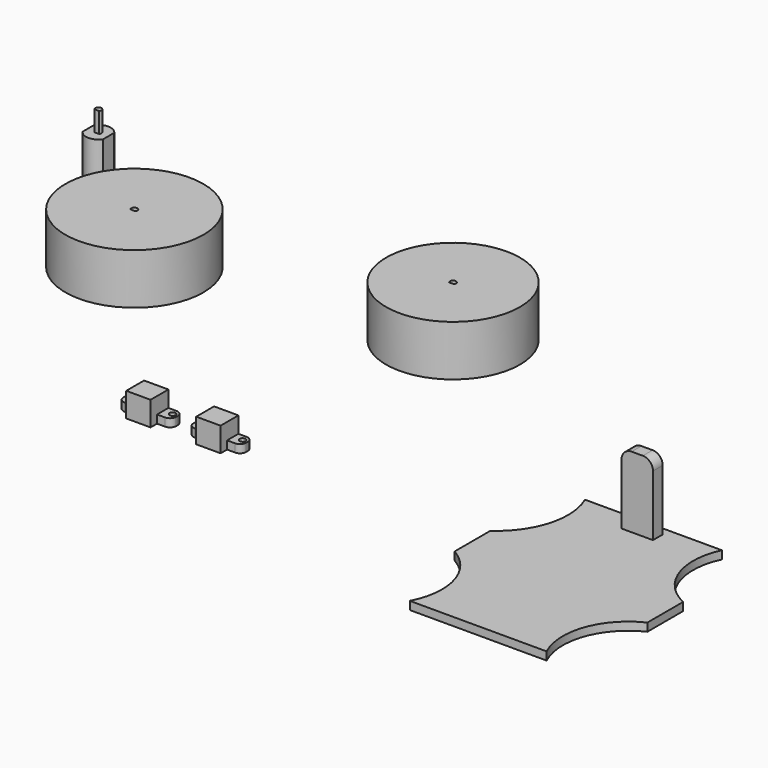
from build123d import *

# Parameters (mm, degrees)
F0_R      = 34
F1_DEPTH  = 25
F4_DEPTH  = 44
F5_DEPTH  = 25
F7_DEPTH  = 10
F8_R      = 33
F9_DEPTH  = 25
F11_DEPTH = 28.1
F13_W     = 95
F13_H     = 108
F14_DEPTH = 4
F16_DEPTH = 25
F17_W     = 15.5
F17_H     = 6
F18_DEPTH = 35
F19_R     = 5
F21_DEPTH = 12
F22_W     = 7
F22_H     = 7
F23_DEPTH = 8
F24_R     = 3
F26_R     = 1.5
F25_R     = 1.5
F27_DEPTH = 25
F29_DEPTH = 12
F30_W     = 7
F30_H     = 7
F31_DEPTH = 8
F32_R     = 3
F33_R     = 3
F34_R     = 1.5
F35_R     = 1.5
F36_DEPTH = 25


with BuildPart() as f1:
    # F0 (on Top) → F1 (new body)
    with BuildSketch(Plane.XY):
        Circle(F0_R)
    extrude(amount=F1_DEPTH)

    # F3 (on face) → F4 (cut)
    with BuildSketch(Plane.XY.offset(25)):
        with BuildLine():
            Line((0, -1), (1.1180339887, -1))
            ThreePointArc((1.1180339887, -1), (0, 1.5), (-1.1180339887, -1))
            Line((-1.1180339887, -1), (0, -1))
        make_face()
    extrude(amount=-F4_DEPTH, mode=Mode.SUBTRACT)


with BuildPart() as f5:
    # F2 (on Top) → F5 (new body)
    with BuildSketch(Plane.XY):
        with BuildLine():
            Line((-56.0500432012, 44.9939276846), (-56.0500432012, 38.1657885869))
            ThreePointArc((-56.0500432012, 38.1657885869), (-50.9907110945, 35.4763581357), (-45.9313789879, 38.1657885869))
            Line((-45.9313789879, 38.1657885869), (-45.9313789879, 44.9939276846))
            ThreePointArc((-45.9313789879, 44.9939276846), (-50.9907110945, 47.6833581357), (-56.0500432012, 44.9939276846))
        make_face()
    extrude(amount=F5_DEPTH)

    # F6 (on face) → F7 (join)
    with BuildSketch(Plane.XY.offset(25)):
        with BuildLine():
            Line((-51.0072966267, 40.5797664396), (-49.872759128, 40.5797664396))
            ThreePointArc((-49.872759128, 40.5797664396), (-50.9907110945, 43.0798581357), (-52.108663061, 40.5797664396))
            Line((-52.108663061, 40.5797664396), (-51.0072966267, 40.5797664396))
        make_face()
    extrude(amount=F7_DEPTH)


with BuildPart() as f9:
    # F8 (on Top) → F9 (new body)
    with BuildSketch(Plane.XY):
        with Locations((133.7766498327, 29.1395578533)):
            Circle(F8_R)
    extrude(amount=F9_DEPTH)

    # F10 (on face) → F11 (cut)
    with BuildSketch(Plane.XY.offset(25)):
        with BuildLine():
            Line((133.7687078238, 28.139536828), (134.8946650155, 28.139536828))
            ThreePointArc((134.8946650155, 28.139536828), (133.7766498327, 30.6395578533), (132.6586346499, 28.139536828))
            Line((132.6586346499, 28.139536828), (133.7687078238, 28.139536828))
        make_face()
    extrude(amount=-F11_DEPTH, mode=Mode.SUBTRACT)


with BuildPart() as f12_1:
    # F12: instance of F5
    add(f5.part.mirror(Plane.XY))


with BuildPart() as f14:
    # F13 (on Top) → F14 (new body)
    with BuildSketch(Plane.XY):
        with Locations((296.7195218801, -103.1332481652)):
            Rectangle(F13_W, F13_H)
    extrude(amount=F14_DEPTH)

    # F15 (on face) → F16 (cut)
    with BuildSketch(Plane.XY.offset(4)):
        with BuildLine():
            Line((261.4695218801, -49.1332481652), (249.2195218801, -49.1332481652))
            Line((249.2195218801, -49.1332481652), (249.2195218801, -92.1332481652))
            ThreePointArc((249.2195218801, -92.1332481652), (263.0342636127, -72.823930403), (261.4695218801, -49.1332481652))
        make_face()
        with BuildLine():
            Line((344.2195218801, -49.1332481652), (328.9695218801, -49.1332481652))
            ThreePointArc((328.9695218801, -49.1332481652), (327.6845782047, -73.7931700502), (344.2195218801, -92.1332481652))
            Line((344.2195218801, -92.1332481652), (344.2195218801, -49.1332481652))
        make_face()
        with BuildLine():
            ThreePointArc((344.2195218801, -114.1332481652), (327.6845782047, -132.4733262803), (328.9695218801, -157.1332481652))
            Line((328.9695218801, -157.1332481652), (344.2195218801, -157.1332481652))
            Line((344.2195218801, -157.1332481652), (344.2195218801, -114.1332481652))
        make_face()
        with BuildLine():
            ThreePointArc((261.4695218801, -157.1332481652), (264.005628305, -133.1658399396), (249.2195218801, -114.1332481652))
            Line((249.2195218801, -114.1332481652), (249.2195218801, -157.1332481652))
            Line((249.2195218801, -157.1332481652), (261.4695218801, -157.1332481652))
        make_face()
    extrude(amount=-F16_DEPTH, mode=Mode.SUBTRACT)

    # F17 (on face) → F18 (join)
    with BuildSketch(Plane.XY.offset(4)):
        with Locations((295.2195218801, -56.1332481652)):
            Rectangle(F17_W, F17_H)
    extrude(amount=F18_DEPTH)

    # F19
    f19_edges = [f14.edges().sort_by_distance(p)[0] for p in [
        (287.469522, -56.133248, 39),
        (302.969522, -56.133248, 39),
    ]]
    fillet(f19_edges, radius=F19_R)


with BuildPart() as f21:
    # F20 (on Top) → F21 (new body)
    with BuildSketch(Plane.XY):
        Polygon((76.4376826286, -96.5886867642), (76.4376826286, -100.5886867642), (88.4376826286, -100.5886867642), (88.4376826286, -96.5886867642), (95.4376826286, -96.5886867642), (95.4376826286, -89.5886867642), (69.4376826286, -89.5886867642), (69.4376826286, -96.5886867642), align=None)
    extrude(amount=F21_DEPTH)

    # F22 (on face) → F23 (cut)
    with BuildSketch(Plane.XY.offset(12)):
        with Locations((91.9376826286, -93.0886867642)):
            Rectangle(F22_W, F22_H)
        with Locations((72.9376826286, -93.0886867642)):
            Rectangle(F22_W, F22_H)
    extrude(amount=-F23_DEPTH, mode=Mode.SUBTRACT)

    # F24
    f24_edges = [f21.edges().sort_by_distance(p)[0] for p in [
        (95.437683, -89.588687, 2),
        (95.437683, -96.588687, 2),
        (69.437683, -96.588687, 2),
        (69.437683, -89.588687, 2),
    ]]
    fillet(f24_edges, radius=F24_R)

    # F26 (on face) + F25 (on face) → F27 (cut)
    with BuildSketch(Plane.XY.offset(4)):
        with Locations((71.9376826286, -92.5886867642)):
            Circle(F26_R)
    with BuildSketch(Plane.XY.offset(4)):
        with Locations((92.9376826286, -92.5886867642)):
            Circle(F25_R)
    extrude(amount=-F27_DEPTH, mode=Mode.SUBTRACT)


with BuildPart() as f29:
    # F28 (on Top) → F29 (new body)
    with BuildSketch(Plane.XY):
        Polygon((110.9677634835, -96.5990356207), (110.9677634835, -100.5990356207), (122.9677634835, -100.5990356207), (122.9677634835, -96.5990356207), (129.9677634835, -96.5990356207), (129.9677634835, -89.5990356207), (103.9677634835, -89.5990356207), (103.9677634835, -96.5990356207), align=None)
    extrude(amount=F29_DEPTH)

    # F30 (on face) → F31 (cut)
    with BuildSketch(Plane.XY.offset(12)):
        with Locations((126.4677634835, -93.0990356207)):
            Rectangle(F30_W, F30_H)
        with Locations((107.4677634835, -93.0990356207)):
            Rectangle(F30_W, F30_H)
    extrude(amount=-F31_DEPTH, mode=Mode.SUBTRACT)

    # F32
    f32_edges = [f29.edges().sort_by_distance(p)[0] for p in [
        (129.967763, -89.599036, 2),
        (129.967763, -96.599036, 2),
    ]]
    fillet(f32_edges, radius=F32_R)

    # F33
    f33_edges = [f29.edges().sort_by_distance(p)[0] for p in [
        (103.967763, -96.599036, 2),
        (103.967763, -89.599036, 2),
    ]]
    fillet(f33_edges, radius=F33_R)

    # F34 (on face) + F35 (on face) → F36 (cut)
    with BuildSketch(Plane.XY.offset(4)):
        with Locations((106.4677634835, -92.5990356207)):
            Circle(F34_R)
    with BuildSketch(Plane.XY.offset(4)):
        with Locations((127.4677634835, -92.5990356207)):
            Circle(F35_R)
    extrude(amount=-F36_DEPTH, mode=Mode.SUBTRACT)


solid = Compound([f1.part, f5.part, f9.part, f12_1.part, f14.part, f21.part, f29.part])
